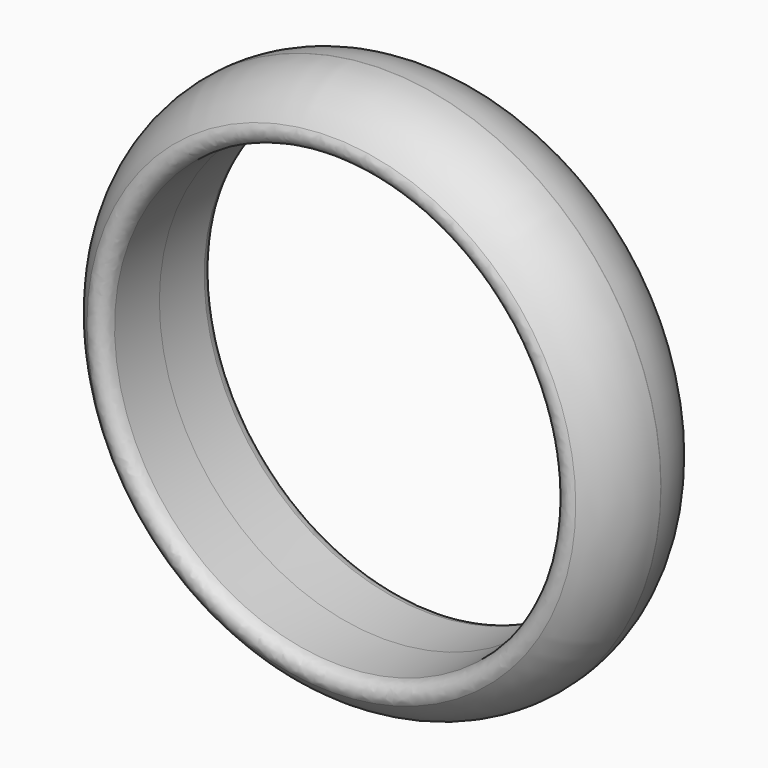
from build123d import *

# Parameters (mm, degrees)
F0_R     = 11.43
F0_R_2   = 9.271
F1_DEPTH = 3.175
F3_R     = 0.508


# Not quite as in the source:
# - a fillet or chamfer that OpenCascade refuses, or shapes differently, is made with other operations: its cross-section is extruded or revolved along the edge and cut away or added


with BuildPart() as f1:
    # F0 (on Front) → F1 (new body)
    with BuildSketch(Plane.XZ):
        Circle(F0_R)
        Circle(F0_R_2, mode=Mode.SUBTRACT)
    extrude(amount=F1_DEPTH)

    # F2: fillet of radius 3.4036 on 1 edges, made by hand

    # F2_s1 → F2_t2 (revolve, cut)
    with BuildSketch(Plane.XY):
        with BuildLine():
            ThreePointArc((11.43, -0.0071199833), (10.8389267572, -1.9239366673), (9.271, -3.175))
            Line((9.271, -3.175), (9.295892, -3.2383576003))
            ThreePointArc((9.295892, -3.2383576003), (10.3505, -3.243072), (11.43, -3.243072))
            Line((11.43, -3.243072), (11.498072, -3.175))
            Line((11.498072, -3.175), (11.498072, -0.0071199833))
            Line((11.498072, -0.0071199833), (11.43, -0.0071199833))
        make_face()
    revolve(axis=Axis((0, -3.175, 0), (0, -1, 0)), mode=Mode.SUBTRACT)

    # F3
    f3_edges = [f1.edges().sort_by_distance(p)[0] for p in [
        (-9.271, -3.175, 0),
    ]]
    fillet(f3_edges, radius=F3_R)

    # F4: F1 across plane


with BuildPart() as f1_1:
    add(f1.part)
    add(f1.part.mirror(Plane.XZ))


solid = f1_1.part
